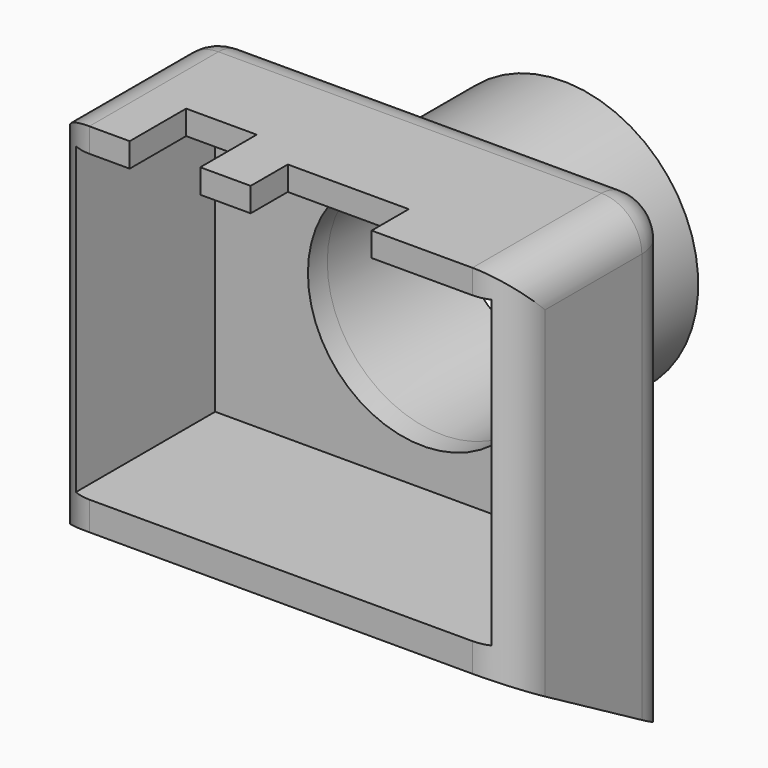
from build123d import *

# Parameters (mm, degrees)
F0_W          = 23
F0_H          = 17.5
F1_DEPTH      = 10
F2_T          = -1.2
F3_R          = 5.7
F4_DEPTH      = 3
F3_R_2        = 6.7
F5_DEPTH      = 7.5
F6_W          = 6
F6_H          = 2.3
F6_W_2        = 3.5
F6_H_2        = 3.5
F7_DEPTH      = 4
F8_DEPTH      = 6
F10_DEPTH     = 30
F11_T1_DEPTH  = 19
F11_T3_DEPTH  = 26.5
F11_T5_DEPTH  = 13
F11_T7_DEPTH  = 27.7264973081
F11_S11_W     = 2
F11_S11_H     = 2
F11_T12_DEPTH = 2
F11_S17_W     = 2
F11_S17_H     = 2
F11_T18_DEPTH = 2


# Not quite as in the source:
# - a fillet or chamfer that OpenCascade refuses, or shapes differently, is made with other operations: its cross-section is extruded or revolved along the edge and cut away or added


with BuildPart() as f1:
    # F0 (on Front) → F1 (new body)
    with BuildSketch(Plane.XZ):
        Rectangle(F0_W, F0_H)
    extrude(amount=F1_DEPTH)

    # F2
    f2_openings = [f1.faces().sort_by_distance(p)[0] for p in [
        (0, -10, 0),
    ]]
    offset(amount=F2_T, openings=f2_openings)

    # F3 (on face) → F4 (cut)
    with BuildSketch(Plane(origin=(0, 0, 0), x_dir=(-1, 0, 0), z_dir=(0, 1, 0))):
        Circle(F3_R)
    extrude(amount=-F4_DEPTH, mode=Mode.SUBTRACT)

    # F3 (on face) → F5 (join)
    with BuildSketch(Plane(origin=(0, 0, 0), x_dir=(-1, 0, 0), z_dir=(0, 1, 0))):
        Circle(F3_R_2)
        Circle(F3_R, mode=Mode.SUBTRACT)
    extrude(amount=F5_DEPTH)

    # F6 (on face) → F7 (cut)
    with BuildSketch(Plane.XY.offset(8.75)):
        with Locations((1.5, -8.85)):
            Rectangle(F6_W, F6_H)
        with Locations((-5.75, -8.25)):
            Rectangle(F6_W_2, F6_H_2)
    extrude(amount=-F7_DEPTH, mode=Mode.SUBTRACT)

    # F8 (add): a face of the model
    f8_faces = [f1.faces().sort_by_distance(p)[0] for p in [
        (0, -5, -8.75),
    ]]
    extrude(f8_faces, amount=F8_DEPTH)

    # F9 (on face) → F10 (cut)
    with BuildSketch(Plane.YZ.offset(11.5)):
        Polygon((-10, -14.75), (0, -14.75), (-10, -8.9764973081), align=None)
    extrude(amount=-F10_DEPTH, mode=Mode.SUBTRACT)

    # F11: fillet of radius 2 on 7 edges, made by hand

    # F11_s2 → F11_t1 (cut)
    with BuildSketch(Plane.YZ.offset(-9.5)):
        with BuildLine():
            ThreePointArc((0, 6.75), (-0.5857864376, 8.1642135624), (-2, 8.75))
            Line((-2, 8.75), (0, 8.75))
            Line((0, 8.75), (0, 6.75))
        make_face()
    extrude(amount=F11_T1_DEPTH, mode=Mode.SUBTRACT)

    # F11_s4 → F11_t3 (cut)
    with BuildSketch(Plane.XY.offset(-19.75)):
        with BuildLine():
            ThreePointArc((-11.5, -2), (-10.9142135624, -0.5857864376), (-9.5, 0))
            Line((-9.5, 0), (-11.5, 0))
            Line((-11.5, 0), (-11.5, -2))
        make_face()
        with BuildLine():
            ThreePointArc((9.5, 0), (10.9142135624, -0.5857864376), (11.5, -2))
            Line((11.5, -2), (11.5, 0))
            Line((11.5, 0), (9.5, 0))
        make_face()
    extrude(amount=F11_T3_DEPTH, mode=Mode.SUBTRACT)

    # F11_s6 → F11_t5 (cut)
    with BuildSketch(Plane.XZ.offset(2)):
        with BuildLine():
            ThreePointArc((9.5, 8.75), (10.9142135624, 8.1642135624), (11.5, 6.75))
            Line((11.5, 6.75), (11.5, 8.75))
            Line((11.5, 8.75), (9.5, 8.75))
        make_face()
        with BuildLine():
            ThreePointArc((-11.5, 6.75), (-10.9142135624, 8.1642135624), (-9.5, 8.75))
            Line((-9.5, 8.75), (-11.5, 8.75))
            Line((-11.5, 8.75), (-11.5, 6.75))
        make_face()
    extrude(amount=F11_T5_DEPTH, mode=Mode.SUBTRACT)

    # F11_s8 → F11_t7 (cut)
    with BuildSketch(Plane.XY.offset(-13.9764973081)):
        with BuildLine():
            ThreePointArc((-11.5, -8), (-10.9142135624, -9.4142135624), (-9.5, -10))
            Line((-9.5, -10), (-11.5, -10))
            Line((-11.5, -10), (-11.5, -8))
        make_face()
        with BuildLine():
            ThreePointArc((9.5, -10), (10.9142135624, -9.4142135624), (11.5, -8))
            Line((11.5, -8), (11.5, -10))
            Line((11.5, -10), (9.5, -10))
        make_face()
    extrude(amount=F11_T7_DEPTH, mode=Mode.SUBTRACT)


with BuildPart() as f11_tool10:
    # F11_s11 → F11_t12 (new body)
    with BuildSketch(Plane.XZ.offset(2)):
        with Locations((10.5, 7.75)):
            Rectangle(F11_S11_W, F11_S11_H)
    extrude(amount=-F11_T12_DEPTH)

    # F11_s13 → F11_t14 (revolve, cut)
    with BuildSketch(Plane(origin=(9.5, -2, 6.75), x_dir=(-0.7071067812, 0, -0.7071067812), z_dir=(0.7071067812, 0, -0.7071067812))):
        with BuildLine():
            ThreePointArc((0, -2), (2, 0), (0, 2))
            Line((0, 2), (0, -2))
        make_face()
    revolve(axis=Axis((9.5, -2, 6.75), (0, 1, 0)), mode=Mode.SUBTRACT)


with BuildPart() as f1_1:
    add(f1.part)

    # F11_t9: cut F11_tool10
    add(f11_tool10.part, mode=Mode.SUBTRACT)


with BuildPart() as f11_tool16:
    # F11_s17 → F11_t18 (new body)
    with BuildSketch(Plane.YZ.offset(-9.5)):
        with Locations((-1, 7.75)):
            Rectangle(F11_S17_W, F11_S17_H)
    extrude(amount=-F11_T18_DEPTH)

    # F11_s19 → F11_t20 (revolve, cut)
    with BuildSketch(Plane(origin=(-9.5, -2, 6.75), x_dir=(0, -0.7071067812, -0.7071067812), z_dir=(0, 0.7071067812, -0.7071067812))):
        with BuildLine():
            ThreePointArc((0, -2), (2, 0), (0, 2))
            Line((0, 2), (0, -2))
        make_face()
    revolve(axis=Axis((-9.5, -2, 6.75), (-1, 0, 0)), mode=Mode.SUBTRACT)


with BuildPart() as f1_2:
    add(f1_1.part)

    # F11_t15: cut F11_tool16
    add(f11_tool16.part, mode=Mode.SUBTRACT)


solid = f1_2.part
